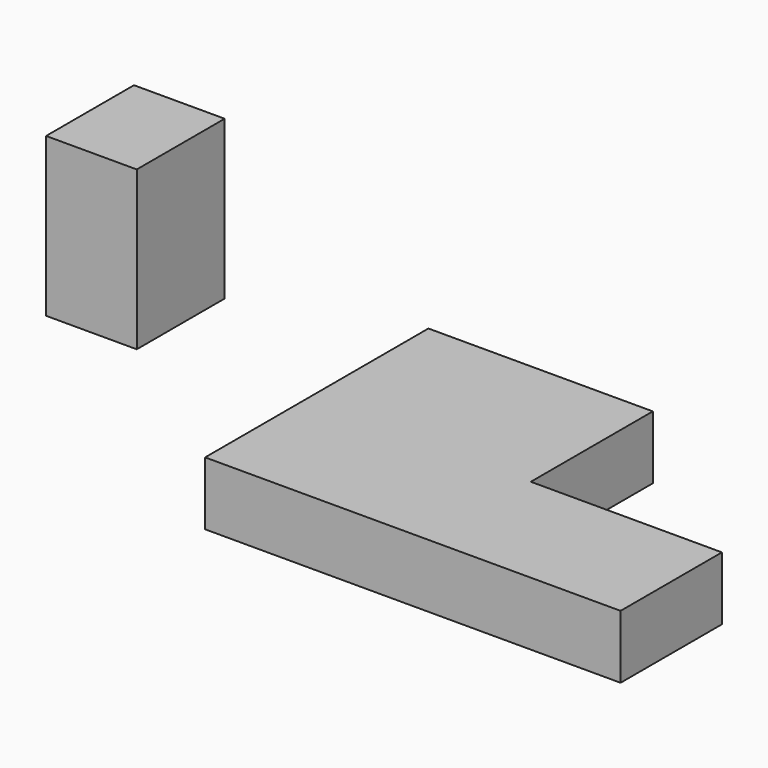
from build123d import *

# Parameters (mm, degrees)
F2_DEPTH = 10
F3_W     = 14.3181830645
F3_H     = 17.3431523144
F4_DEPTH = 25


# Not quite as in the source:
# - a feature names something its author has since deleted; it is built from what else it names


with BuildPart() as f2:
    # F0 (on Top) → F2 (new body)
    with BuildSketch(Plane.XY):
        Polygon((0, 44.0678059284), (0, 0), (65.5932351728, 0), (65.5932351728, 20), (35.4237365217, 20), (35.4237365217, 44.0678059284), align=None)
    extrude(amount=F2_DEPTH)


with BuildPart() as f4:
    # F3 (on Top) → F4 (new body)
    with BuildSketch(Plane.XY):
        with Locations((-43.7612049282, 40.9379024059)):
            Rectangle(F3_W, F3_H)
    extrude(amount=F4_DEPTH)


solid = Compound([f2.part, f4.part])
